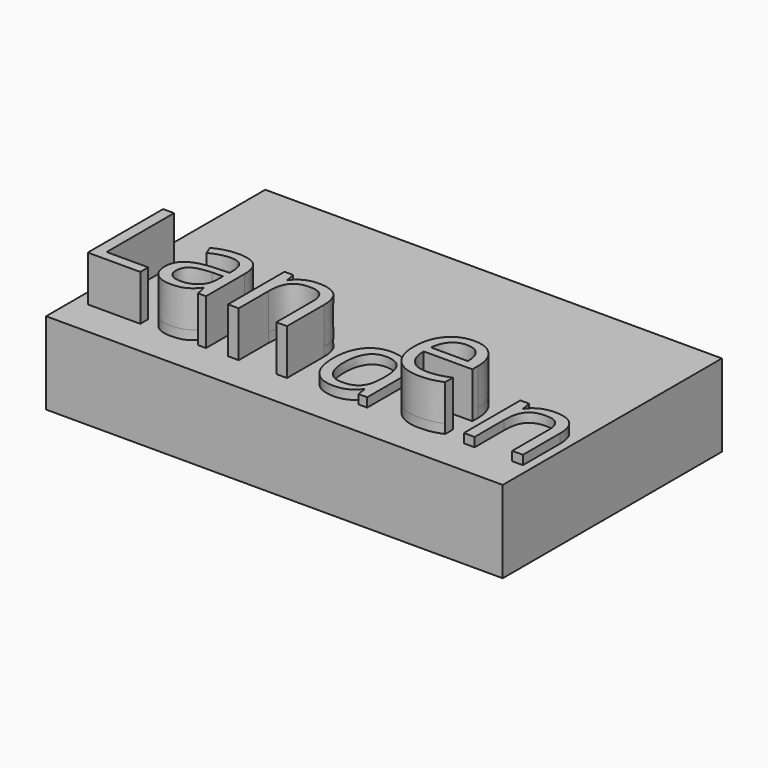
from build123d import *

# Parameters (mm, degrees)
F0_W         = 63.5
F0_H         = 38.1
F1_DEPTH     = 6.35
F2_TEXT_SIZE = 18.3476297968
F3_DEPTH     = 6.35
F4_DEPTH     = 5.08
F5_DEPTH     = 5.08


# Not quite as in the source:
# - Text() gives the source's letters only with a copy of the font that has no kerning and outlines rounded to 1/6400 em; it was checked with that copy


with BuildPart() as f1:
    # F0 (on Top) → F1 (new body)
    with BuildSketch(Plane.XY):
        with Locations((31.75, 19.05)):
            Rectangle(F0_W, F0_H)
    extrude(amount=F1_DEPTH)

    # F2 (on face) → F3 (join)
    with BuildSketch(Plane.XY.offset(6.35)):
        with Locations((0, 4.997215051)):
            Text('Landen', F2_TEXT_SIZE, font='Open Sans', text_align=(TextAlign.LEFT, TextAlign.BOTTOM))
    extrude(amount=F3_DEPTH)

    # F2 (on face) → F4 (join)
    with BuildSketch(Plane.XY.offset(6.35)):
        with Locations((0, 4.997215051)):
            Text('Landen', F2_TEXT_SIZE, font='Open Sans', text_align=(TextAlign.LEFT, TextAlign.BOTTOM))
    extrude(amount=F4_DEPTH)

    # F5 (add): faces of the model
    f5_faces = [f1.faces().sort_by_distance(p)[0] for p in [
        (3.1726789495, 12.2359283693, 12.7),
        (17.1159679109, 5.7232654285, 12.7),
        (31.6499719856, 20.2327347678, 6.35),
        (28.1525036401, 8.1736484596, 12.7),
        (36.3841564332, 9.8900430816, 6.35),
        (47.1833043847, 10.0497131266, 12.7),
    ]]
    extrude(f5_faces, amount=F5_DEPTH)


solid = f1.part
